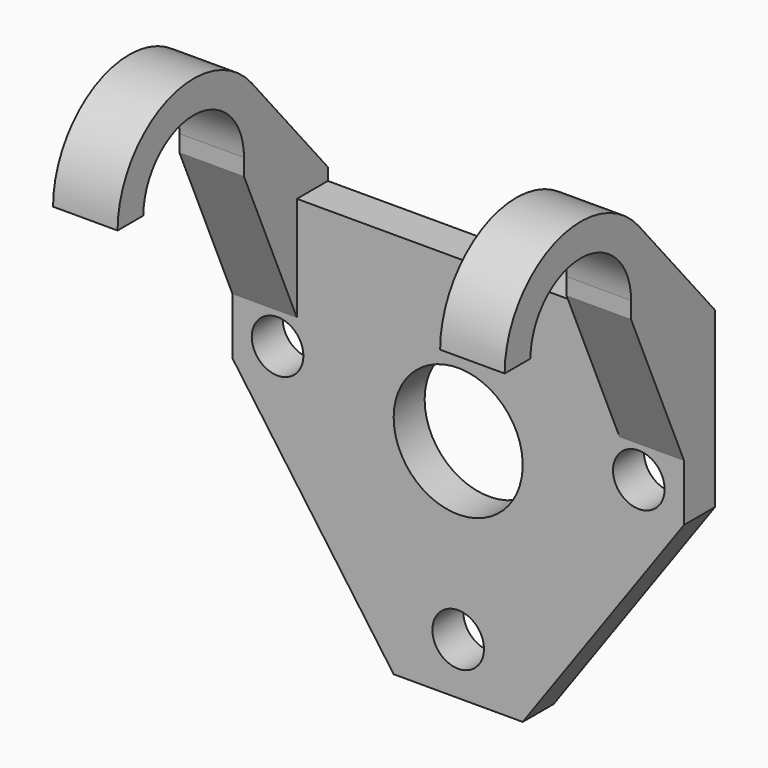
from build123d import *

# Parameters (mm, degrees)
F1_DEPTH  = 70
F4_W      = 50
F4_H      = 24.5480843189
F5_DEPTH  = 25
F7_DEPTH  = 40.7510000745
F8_R      = 10
F9_DEPTH  = 40.7510000745
F10_R     = 6.38
F11_DEPTH = 40.7510000745
F6_R      = 4
F12_DEPTH = 40.7510000745
F15_DEPTH = 10
F16_R     = 4
F17_DEPTH = 40.7510000745
F19_DEPTH = 10


# Not quite as in the source:
# - a pattern or mirror of a feature is missing from the dataset's text; its kind, count and spacing are read off the source's solid


with BuildPart() as f1:
    # F0 (on Right) → F1 (new body)
    with BuildSketch(Plane.YZ):
        with BuildLine():
            ThreePointArc((-9.75, 0), (0, 9.75), (9.75, 0))
            Line((9.75, 0), (9.75, -2.5980842444))
            Line((9.75, -2.5980842444), (20, -9.7980842444))
            Line((20, -9.7980842444), (20, -69.7980842444))
            Line((20, -69.7980842444), (26, -69.7980842444))
            Line((26, -69.7980842444), (26, -7.9024389721))
            Line((26, -7.9024389721), (14.7500000745, 0))
            ThreePointArc((14.7500000745, 0), (0, 14.7500000745), (-14.7500000745, 0))
            Line((-14.7500000745, 0), (-9.75, 0))
        make_face()
    extrude(amount=F1_DEPTH)

    # F4 (on face) → F5 (cut)
    with BuildSketch(Plane(origin=(0, 26, 0), x_dir=(-1, 0, 0), z_dir=(0, 1, 0))):
        Polygon((-45, -69.7980842444), (-70, -34.7980842444), (-90, -34.7980842444), (-90, -94.7980842444), (20, -94.7980842444), (20, -34.7980842444), (0, -34.7980842444), (-25, -69.7980842444), align=None)
        with Locations((-35, 2.475957915)):
            Rectangle(F4_W, F4_H)
    extrude(amount=-F5_DEPTH, mode=Mode.SUBTRACT)

    # F4 (on face) → F7 (cut, through all)
    with BuildSketch(Plane(origin=(0, 26, 0), x_dir=(-1, 0, 0), z_dir=(0, 1, 0))):
        Polygon((-45, -69.7980842444), (-70, -34.7980842444), (-90, -34.7980842444), (-90, -94.7980842444), (20, -94.7980842444), (20, -34.7980842444), (0, -34.7980842444), (-25, -69.7980842444), align=None)
        with Locations((-35, 2.475957915)):
            Rectangle(F4_W, F4_H)
    extrude(amount=-F7_DEPTH, mode=Mode.SUBTRACT)

    # F8 (on face) → F9 (cut, through all)
    with BuildSketch(Plane(origin=(0, 26, 0), x_dir=(-1, 0, 0), z_dir=(0, 1, 0))):
        with Locations((-35, -34.7424389721)):
            Circle(F8_R)
    extrude(amount=-F9_DEPTH, mode=Mode.SUBTRACT)

    # F10 (on face) → F11 (cut, through all)
    with BuildSketch(Plane(origin=(0, 26, 0), x_dir=(-1, 0, 0), z_dir=(0, 1, 0))):
        with Locations((-35, -34.7424389721)):
            Circle(F10_R)
    extrude(amount=-F11_DEPTH, mode=Mode.SUBTRACT)

    # F6 (on face) → F12 (cut, through all)
    with BuildSketch(Plane(origin=(0, 26, 0), x_dir=(-1, 0, 0), z_dir=(0, 1, 0))):
        with Locations((-63, -30.9024389721)):
            Circle(F6_R)
        with Locations((-7, -30.9024389721)):
            Circle(F6_R)
    extrude(amount=-F12_DEPTH, mode=Mode.SUBTRACT)

    # F14 (on face) → F15 (join)
    with BuildSketch(Plane(origin=(0, 0, 0), x_dir=(0, -1, 0), z_dir=(-1, 0, 0))):
        Polygon((-20, -9.7980842444), (-20, -25.9981378913), (-9.75, -2.5980842444), align=None)
    f15 = extrude(amount=-F15_DEPTH)

    # F15_copies: F15 across plane
    add(f15.mirror(Plane(origin=(35, 0, 0), x_dir=(0, 0, 1), z_dir=(1, 0, 0))))

    # F16 (on face) → F17 (cut, through all)
    with BuildSketch(Plane(origin=(0, 26, 0), x_dir=(-1, 0, 0), z_dir=(0, 1, 0))):
        with Locations((-35, -61.7980842444)):
            Circle(F16_R)
    extrude(amount=-F17_DEPTH, mode=Mode.SUBTRACT)

    # F18 (on face) → F19 (join)
    with BuildSketch(Plane(origin=(0, 0, 0), x_dir=(0, -1, 0), z_dir=(-1, 0, 0))):
        Polygon((-11.2626504483, 9.5244531117), (-26, -7.9024389721), (-14.7500000745, 0), align=None)
    f19 = extrude(amount=-F19_DEPTH)

    # F19_copies: F19 across plane
    add(f19.mirror(Plane(origin=(35, 0, 0), x_dir=(0, 0, 1), z_dir=(1, 0, 0))))


solid = f1.part
